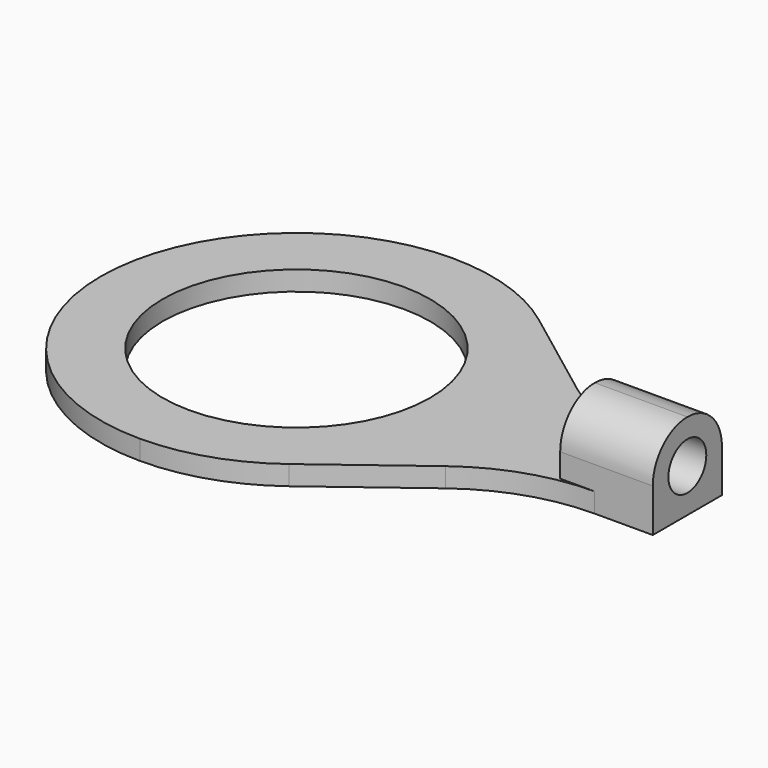
from build123d import *

# Parameters (mm, degrees)
F0_R     = 6.5
F1_DEPTH = 0.95
F3_DEPTH = 3.25
F4_R     = 2.09999
F5_R     = 1.15
F6_DEPTH = 25


# Not quite as in the source:
# - a fillet or chamfer is up to 0.001 mm smaller than in the source, because OpenCascade refuses the exact size


with BuildPart() as f1:
    # F0 (on Top) → F1 (new body)
    with BuildSketch(Plane.XY):
        with BuildLine():
            Line((25.6782327866, 7.4), (28.5, 7.4))
            Line((28.5, 7.4), (28.5, 11.6))
            Line((28.5, 11.6), (25.6782327866, 11.6))
            ThreePointArc((25.6782327866, 11.6), (22.6641990968, 12.0908046465), (19.9615973522, 13.5125050702))
            Line((19.9615973522, 13.5125050702), (15.2166354344, 17.0874949298))
            ThreePointArc((15.2166354344, 17.0874949298), (12.5140336898, 18.5091953535), (9.5, 19))
            ThreePointArc((9.5, 19), (2.7824855787, 16.2175144213), (0, 9.5))
            ThreePointArc((0, 9.5), (2.7824855787, 2.7824855787), (9.5, 0))
            ThreePointArc((9.5, 0), (12.5140336898, 0.4908046465), (15.2166354344, 1.9125050702))
            Line((15.2166354344, 1.9125050702), (19.9615973522, 5.4874949298))
            ThreePointArc((19.9615973522, 5.4874949298), (22.6641990968, 6.9091953535), (25.6782327866, 7.4))
        make_face()
        with Locations((9.5, 9.5)):
            Circle(F0_R, mode=Mode.SUBTRACT)
    extrude(amount=F1_DEPTH)

    # F2 (on face) → F3 (join)
    with BuildSketch(Plane.XY.offset(0.95)):
        Polygon((28.5, 7.4), (28.5, 11.6), (25.6782327866, 11.6), (24, 11.6), (24, 7.4), (25.6782327866, 7.4), align=None)
    extrude(amount=F3_DEPTH)

    # F4 (radius 2.1 in the source; OpenCascade refuses exactly that, so slightly less here)
    f4_edges = [f1.edges().sort_by_distance(p)[0] for p in [
        (26.25, 11.6, 4.2),
        (26.25, 7.4, 4.2),
    ]]
    fillet(f4_edges, radius=F4_R)

    # F5 (on face) → F6 (cut)
    with BuildSketch(Plane.YZ.offset(28.5)):
        with Locations((9.5, 2.1)):
            Circle(F5_R)
    extrude(amount=-F6_DEPTH, mode=Mode.SUBTRACT)


solid = f1.part
